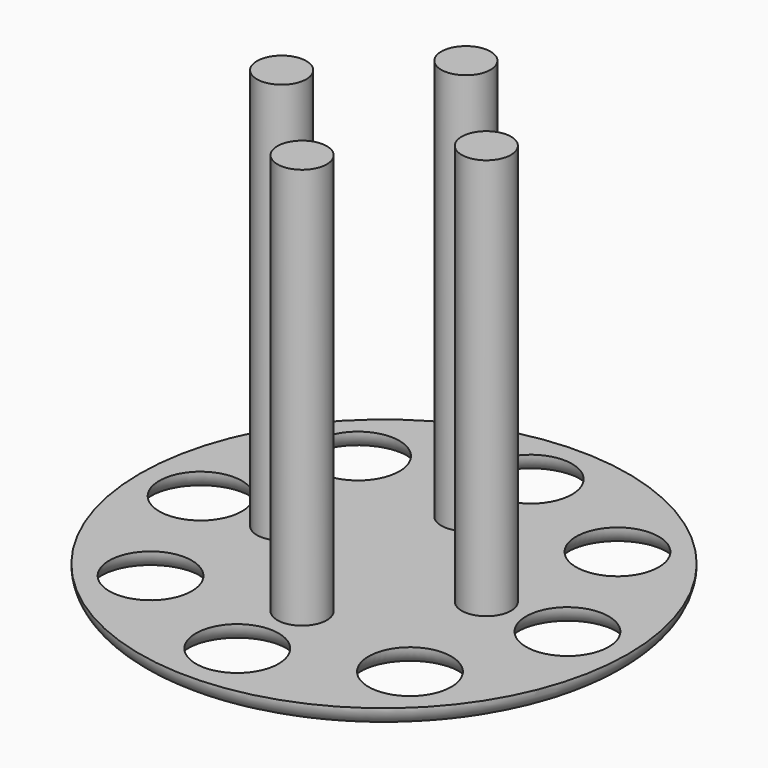
from build123d import *

# Parameters (mm, degrees)
F0_R     = 60.8423289751
F0_R_2   = 10.3008294325
F1_DEPTH = 5
F3_R     = 6.1486808816
F4_DEPTH = 100


# Not quite as in the source:
# - a fillet or chamfer that OpenCascade refuses, or shapes differently, is made with other operations: its cross-section is extruded or revolved along the edge and cut away or added


with BuildPart() as f1:
    # F0 (on Top) → F1 (new body)
    with BuildSketch(Plane.XY):
        Circle(F0_R)
        with Locations((-32.3162567806, -32.3162567806)):
            Circle(F0_R_2, mode=Mode.SUBTRACT)
        with Locations((0, -45.7020886242)):
            Circle(F0_R_2, mode=Mode.SUBTRACT)
        with Locations((32.3162567806, -32.3162567806)):
            Circle(F0_R_2, mode=Mode.SUBTRACT)
        with Locations((-45.7020886242, 0)):
            Circle(F0_R_2, mode=Mode.SUBTRACT)
        with Locations((-32.3162567806, 32.3162567806)):
            Circle(F0_R_2, mode=Mode.SUBTRACT)
        with Locations((45.7020886242, 0)):
            Circle(F0_R_2, mode=Mode.SUBTRACT)
        with Locations((0, 45.7020886242)):
            Circle(F0_R_2, mode=Mode.SUBTRACT)
        with Locations((32.3162567806, 32.3162567806)):
            Circle(F0_R_2, mode=Mode.SUBTRACT)
    extrude(amount=F1_DEPTH)

    # F2: fillet of radius 5.08 on 9 edges, made by hand

    # F2_s1 → F2_t2 (revolve, cut)
    with BuildSketch(Plane.XZ):
        with BuildLine():
            ThreePointArc((60.8423289751, 5.08), (59.3544314235, 1.4878975516), (55.7623289751, 0))
            Line((55.7623289751, 0), (60.8423289751, 0))
            Line((60.8423289751, 0), (60.8423289751, 5.08))
        make_face()
    revolve(axis=Axis((0, 0, 0), (0, 0, 1)), mode=Mode.SUBTRACT)

    # F2_s3 → F2_t4 (revolve, cut)
    with BuildSketch(Plane.XZ.offset(32.3162567806)):
        with BuildLine():
            ThreePointArc((-22.0154273481, 5.08), (-20.5275297965, 1.4878975516), (-16.9354273481, 0))
            Line((-16.9354273481, 0), (-22.0154273481, 0))
            Line((-22.0154273481, 0), (-22.0154273481, 5.08))
        make_face()
    revolve(axis=Axis((-32.3162567806, -32.3162567806, 0), (0, 0, 1)), mode=Mode.SUBTRACT)

    # F2_s5 → F2_t6 (revolve, cut)
    with BuildSketch(Plane.XZ.offset(45.7020886242)):
        with BuildLine():
            ThreePointArc((10.3008294325, 5.08), (11.7887269841, 1.4878975516), (15.3808294325, 0))
            Line((15.3808294325, 0), (10.3008294325, 0))
            Line((10.3008294325, 0), (10.3008294325, 5.08))
        make_face()
    revolve(axis=Axis((0, -45.7020886242, 0), (0, 0, 1)), mode=Mode.SUBTRACT)

    # F2_s7 → F2_t8 (revolve, cut)
    with BuildSketch(Plane.XZ.offset(32.3162567806)):
        with BuildLine():
            ThreePointArc((42.6170862131, 5.08), (44.1049837647, 1.4878975516), (47.6970862131, 0))
            Line((47.6970862131, 0), (42.6170862131, 0))
            Line((42.6170862131, 0), (42.6170862131, 5.08))
        make_face()
    revolve(axis=Axis((32.3162567806, -32.3162567806, 0), (0, 0, 1)), mode=Mode.SUBTRACT)

    # F2_s9 → F2_t10 (revolve, cut)
    with BuildSketch(Plane.XZ):
        with BuildLine():
            ThreePointArc((-35.4012591917, 5.08), (-33.9133616402, 1.4878975516), (-30.3212591917, 0))
            Line((-30.3212591917, 0), (-35.4012591917, 0))
            Line((-35.4012591917, 0), (-35.4012591917, 5.08))
        make_face()
    revolve(axis=Axis((-45.7020886242, 0, 0), (0, 0, 1)), mode=Mode.SUBTRACT)

    # F2_s11 → F2_t12 (revolve, cut)
    with BuildSketch(Plane.XZ.offset(-32.3162567806)):
        with BuildLine():
            ThreePointArc((-22.0154273481, 5.08), (-20.5275297965, 1.4878975516), (-16.9354273481, 0))
            Line((-16.9354273481, 0), (-22.0154273481, 0))
            Line((-22.0154273481, 0), (-22.0154273481, 5.08))
        make_face()
    revolve(axis=Axis((-32.3162567806, 32.3162567806, 0), (0, 0, 1)), mode=Mode.SUBTRACT)

    # F2_s13 → F2_t14 (revolve, cut)
    with BuildSketch(Plane.XZ):
        with BuildLine():
            ThreePointArc((56.0029180567, 5.08), (57.4908156083, 1.4878975516), (61.0829180567, 0))
            Line((61.0829180567, 0), (56.0029180567, 0))
            Line((56.0029180567, 0), (56.0029180567, 5.08))
        make_face()
    revolve(axis=Axis((45.7020886242, 0, 0), (0, 0, 1)), mode=Mode.SUBTRACT)

    # F2_s15 → F2_t16 (revolve, cut)
    with BuildSketch(Plane.XZ.offset(-45.7020886242)):
        with BuildLine():
            ThreePointArc((10.3008294325, 5.08), (11.7887269841, 1.4878975516), (15.3808294325, 0))
            Line((15.3808294325, 0), (10.3008294325, 0))
            Line((10.3008294325, 0), (10.3008294325, 5.08))
        make_face()
    revolve(axis=Axis((0, 45.7020886242, 0), (0, 0, 1)), mode=Mode.SUBTRACT)

    # F2_s17 → F2_t18 (revolve, cut)
    with BuildSketch(Plane.XZ.offset(-32.3162567806)):
        with BuildLine():
            ThreePointArc((42.6170862131, 5.08), (44.1049837647, 1.4878975516), (47.6970862131, 0))
            Line((47.6970862131, 0), (42.6170862131, 0))
            Line((42.6170862131, 0), (42.6170862131, 5.08))
        make_face()
    revolve(axis=Axis((32.3162567806, 32.3162567806, 0), (0, 0, 1)), mode=Mode.SUBTRACT)

    # F3 (on face) → F4 (join)
    with BuildSketch(Plane.XY.offset(5)):
        with Locations((0, 25.5040973425)):
            Circle(F3_R)
        with Locations((-25.5040973425, 0)):
            Circle(F3_R)
        with Locations((0, -25.5040973425)):
            Circle(F3_R)
        with Locations((25.5040973425, 0)):
            Circle(F3_R)
    extrude(amount=F4_DEPTH)


solid = f1.part
